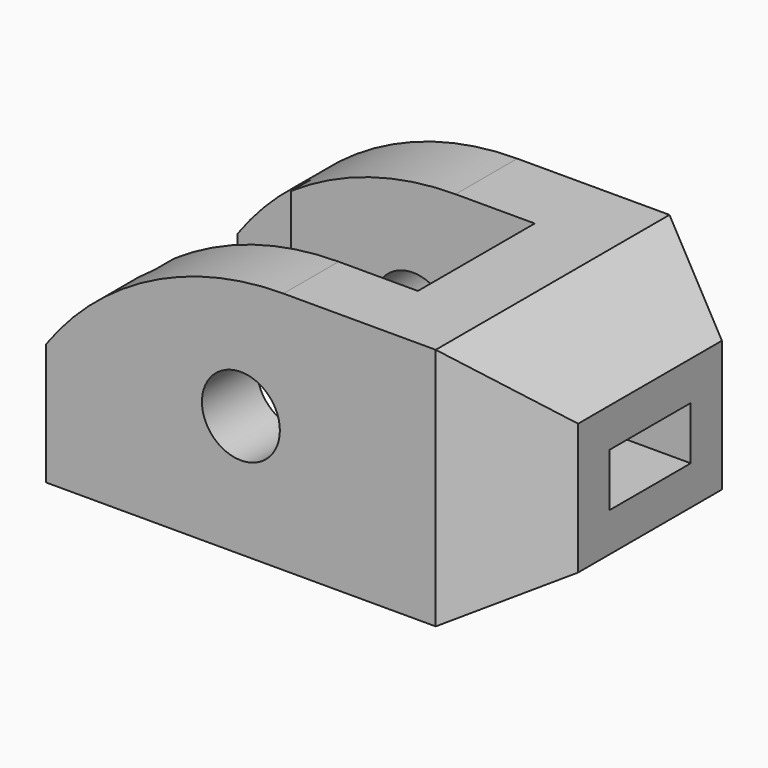
from build123d import *

# Parameters (mm, degrees)
F0_R     = 8
F1_DEPTH = 60
F3_DEPTH = 173
F4_DEPTH = 50.001
F5_W     = 20.9059892324
F5_H     = 10.9059892324
F6_DEPTH = 100.001


# Not quite as in the source:
# - an extrude ends at something that could not be found from the text; its depth is read off the source's solid


with BuildPart() as f1:
    # F0 (on Front) → F1 (new body)
    with BuildSketch(Plane.XZ):
        with BuildLine():
            Line((-76.5279262885, 0), (3.4720737115, 0))
            Line((3.4720737115, 0), (3.4720737115, 50))
            Line((3.4720737115, 50), (-27.7939545645, 50))
            ThreePointArc((-27.7939545645, 50), (-55.1800824397, 43.3853912602), (-76.5279262885, 25))
            Line((-76.5279262885, 25), (-76.5279262885, 0))
        make_face()
        with Locations((-36.5279262885, 25)):
            Circle(F0_R, mode=Mode.SUBTRACT)
        Polygon((3.4720737115, 50), (3.4720737115, 0), (23.4720737115, 11.5470053838), (23.4720737115, 38.4529946162), align=None)
    extrude(amount=F1_DEPTH)

    # F2 (on Top) → F3 (cut, through all)
    with BuildSketch(Plane.XY):
        Polygon((-61.5279262885, -10.8334115148), (-76.5279262885, -10.8334115148), (-76.5279262885, -50.8334115148), (-61.5279262885, -50.8334115148), (-61.5279262885, -45.8334115148), (-11.5279262885, -45.8334115148), (-11.5279262885, -15.8334115148), (-61.5279262885, -15.8334115148), align=None)
        Polygon((23.4720737115, 0), (3.4720737115, 0), (23.4720737115, -11.5470053838), align=None)
        Polygon((23.4720737115, -60), (23.4720737115, -48.4529946162), (3.4720737115, -60), align=None)
    extrude(amount=-F3_DEPTH, mode=Mode.SUBTRACT)

    # F2 (on Top) → F4 (cut, through all)
    with BuildSketch(Plane.XY):
        Polygon((-61.5279262885, -10.8334115148), (-76.5279262885, -10.8334115148), (-76.5279262885, -50.8334115148), (-61.5279262885, -50.8334115148), (-61.5279262885, -45.8334115148), (-11.5279262885, -45.8334115148), (-11.5279262885, -15.8334115148), (-61.5279262885, -15.8334115148), align=None)
        Polygon((23.4720737115, 0), (3.4720737115, 0), (23.4720737115, -11.5470053838), align=None)
        Polygon((23.4720737115, -60), (23.4720737115, -48.4529946162), (3.4720737115, -60), align=None)
    extrude(amount=F4_DEPTH, mode=Mode.SUBTRACT)

    # F5 (on face) → F6 (cut, through all)
    with BuildSketch(Plane.YZ.offset(23.4720737115)):
        with Locations((-30, 25)):
            Rectangle(F5_W, F5_H)
    extrude(amount=-F6_DEPTH, mode=Mode.SUBTRACT)


solid = f1.part
